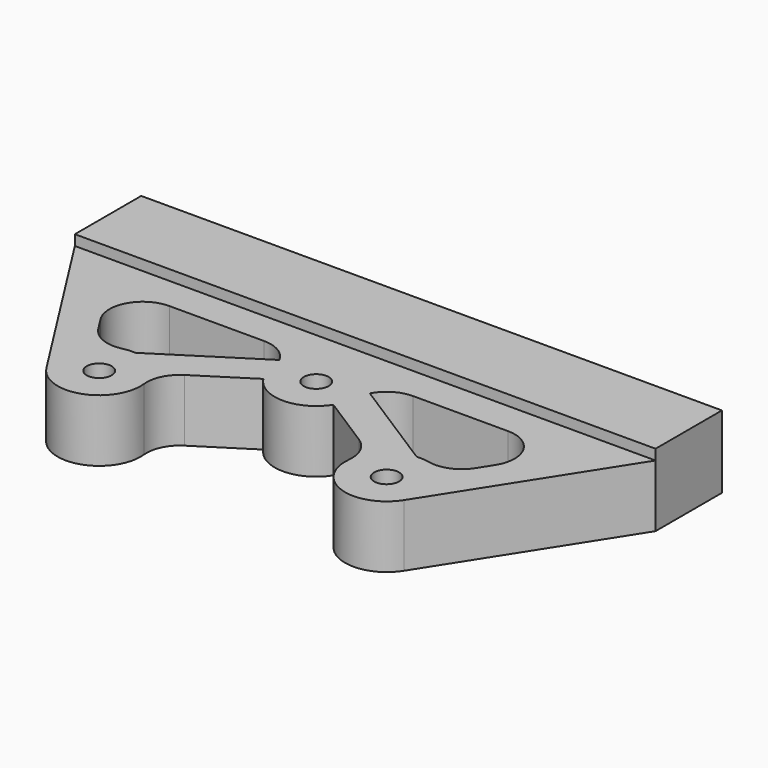
from build123d import *

# Parameters (mm, degrees)
F1_DEPTH       = 9.525
F2_T1_DEPTH    = 9.525
F3_W           = 88.9
F3_H           = 12.7
F4_DEPTH       = 1.5875
F6_D           = 3.81
F6_CSINK_D     = 6.35
F6_CSINK_ANGLE = 60


# Not quite as in the source:
# - a fillet or chamfer that OpenCascade refuses, or shapes differently, is made with other operations: its cross-section is extruded or revolved along the edge and cut away or added


with BuildPart() as f1:
    # F0 (on Top) → F1 (new body)
    with BuildSketch(Plane.XY):
        with BuildLine():
            Line((-16.6466649714, -10.6111378352), (-5.3546547037, -3.4132349764))
            ThreePointArc((-5.3546547037, -3.4132349764), (0, -6.35), (5.3546547037, -3.4132349764))
            Line((5.3546547037, -3.4132349764), (16.6466649714, -10.6111378352))
            ThreePointArc((16.6466649714, -10.6111378352), (18.5880846986, -19.3790275153), (27.3559743788, -17.437607788))
            Line((27.3559743788, -17.437607788), (44.45, 9.3793577389))
            Line((44.45, 9.3793577389), (44.45, 22.0793577389))
            Line((44.45, 22.0793577389), (-44.45, 22.0793577389))
            Line((-44.45, 22.0793577389), (-44.45, 9.3793577389))
            Line((-44.45, 9.3793577389), (-27.3559743788, -17.437607788))
            ThreePointArc((-27.3559743788, -17.437607788), (-18.5880846986, -19.3790275153), (-16.6466649714, -10.6111378352))
        make_face()
        with BuildLine():
            Line((-5.9433808033, 2.2357827771), (-21.519114834, -7.6927080628))
            ThreePointArc((-21.519114834, -7.6927080628), (-24.1573435523, -8.0515961507), (-26.4165242416, -9.4605510978))
            Line((-26.4165242416, -9.4605510978), (-35.1875477179, 4.2993577389))
            Line((-35.1875477179, 4.2993577389), (-4.6731170575, 4.2993577389))
            ThreePointArc((-4.6731170575, 4.2993577389), (-5.4075957794, 3.3287246638), (-5.9433808033, 2.2357827771))
        make_face(mode=Mode.SUBTRACT)
        with BuildLine():
            ThreePointArc((5.9433808033, 2.2357827771), (5.4075957794, 3.3287246638), (4.6731170575, 4.2993577389))
            Line((4.6731170575, 4.2993577389), (35.1875477179, 4.2993577389))
            Line((35.1875477179, 4.2993577389), (26.4165242416, -9.4605510978))
            ThreePointArc((26.4165242416, -9.4605510978), (24.1573435523, -8.0515961507), (21.519114834, -7.6927080628))
            Line((21.519114834, -7.6927080628), (5.9433808033, 2.2357827771))
        make_face(mode=Mode.SUBTRACT)
    extrude(amount=F1_DEPTH)

    # F2: fillet of radius 5.08 on 10 edges, made by hand

    # F2_s2 → F2_t1 (join)
    with BuildSketch(Plane.XY):
        with BuildLine():
            ThreePointArc((25.9250954358, 4.2993577389), (30.3791827129, 1.6622057751), (30.2088191987, -3.5112302422))
            Line((30.2088191987, -3.5112302422), (35.1875477179, 4.2993577389))
            Line((35.1875477179, 4.2993577389), (25.9250954358, 4.2993577389))
        make_face()
        with BuildLine():
            ThreePointArc((28.86470245, -5.6198694424), (26.5021187872, -7.5920062794), (23.4344635706, -7.8382109503))
            ThreePointArc((23.4344635706, -7.8382109503), (25.0359187955, -8.4464064996), (26.4165242416, -9.4605510978))
            Line((26.4165242416, -9.4605510978), (28.86470245, -5.6198694424))
        make_face()
        with BuildLine():
            ThreePointArc((6.3351726778, -0.433690145), (7.9360436505, 2.9321004414), (11.4033108201, 4.2993577389))
            Line((11.4033108201, 4.2993577389), (4.6731170575, 4.2993577389))
            ThreePointArc((4.6731170575, 4.2993577389), (5.9913309283, 2.1039139022), (6.3351726778, -0.433690145))
        make_face()
        with BuildLine():
            ThreePointArc((5.4870763048, 3.1960121441), (6.2133994477, 2.2333964199), (7.1461493675, 1.4690980964))
            Line((7.1461493675, 1.4690980964), (5.9433808033, 2.2357827771))
            ThreePointArc((5.9433808033, 2.2357827771), (5.7353594076, 2.7254637156), (5.4870763048, 3.1960121441))
        make_face()
        with BuildLine():
            ThreePointArc((-7.1461493675, 1.4690980964), (-6.2133994477, 2.2333964199), (-5.4870763048, 3.1960121441))
            ThreePointArc((-5.4870763048, 3.1960121441), (-5.7353594076, 2.7254637156), (-5.9433808033, 2.2357827771))
            Line((-5.9433808033, 2.2357827771), (-7.1461493675, 1.4690980964))
        make_face()
        with BuildLine():
            ThreePointArc((-11.4033108201, 4.2993577389), (-7.9360436505, 2.9321004414), (-6.3351726778, -0.433690145))
            ThreePointArc((-6.3351726778, -0.433690145), (-5.9913309283, 2.1039139022), (-4.6731170575, 4.2993577389))
            Line((-4.6731170575, 4.2993577389), (-11.4033108201, 4.2993577389))
        make_face()
        with BuildLine():
            ThreePointArc((-23.4344635706, -7.8382109503), (-26.5021187872, -7.5920062794), (-28.86470245, -5.6198694424))
            Line((-28.86470245, -5.6198694424), (-26.4165242416, -9.4605510978))
            ThreePointArc((-26.4165242416, -9.4605510978), (-25.0359187955, -8.4464064996), (-23.4344635706, -7.8382109503))
        make_face()
        with BuildLine():
            ThreePointArc((-30.2088191987, -3.5112302422), (-30.3791827129, 1.6622057751), (-25.9250954358, 4.2993577389))
            Line((-25.9250954358, 4.2993577389), (-35.1875477179, 4.2993577389))
            Line((-35.1875477179, 4.2993577389), (-30.2088191987, -3.5112302422))
        make_face()
        with BuildLine():
            ThreePointArc((-15.6875923106, -13.3466215538), (-15.2148846453, -10.6031015998), (-13.3671984002, -8.5206967846))
            Line((-13.3671984002, -8.5206967846), (-16.6466649714, -10.6111378352))
            ThreePointArc((-16.6466649714, -10.6111378352), (-16.0089492913, -11.9234213166), (-15.6875923106, -13.3466215538))
        make_face()
        with BuildLine():
            ThreePointArc((13.3671984002, -8.5206967846), (15.2148846453, -10.6031015998), (15.6875923106, -13.3466215538))
            ThreePointArc((15.6875923106, -13.3466215538), (16.0089492913, -11.9234213166), (16.6466649714, -10.6111378352))
            Line((16.6466649714, -10.6111378352), (13.3671984002, -8.5206967846))
        make_face()
    extrude(amount=F2_T1_DEPTH)

    # F3 (on face) → F4 (join)
    with BuildSketch(Plane.XY.offset(9.525)):
        with Locations((0, 15.7293577389)):
            Rectangle(F3_W, F3_H)
    extrude(amount=F4_DEPTH)

    # F6 (through all)
    with Locations(Plane(origin=(0, 0, 0), x_dir=(1, 0, 0), z_dir=(0, 0, -1))):
        with Locations((0, 0), (-22.0013196751, 14.0243728116), (22.0013196751, 14.0243728116)):
            CounterSinkHole(F6_D / 2, F6_CSINK_D / 2, counter_sink_angle=F6_CSINK_ANGLE)


solid = f1.part
